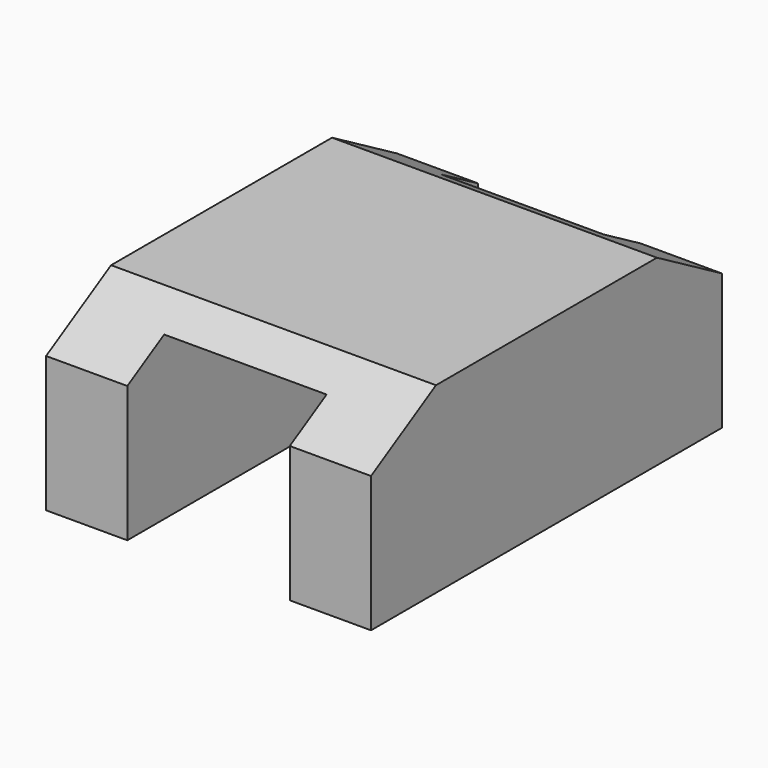
from build123d import *

# Parameters (mm, degrees)
F1_DEPTH    = 68.58
F2_T1_DEPTH = 116.511978168


# Not quite as in the source:
# - a fillet or chamfer that OpenCascade refuses, or shapes differently, is made with other operations: its cross-section is extruded or revolved along the edge and cut away or added


with BuildPart() as f1:
    # F0 (on Front) → F1 (new body)
    with BuildSketch(Plane.XZ):
        Polygon((-12.7, 0), (0, 0), (0, 28.575), (-50.8, 28.575), (-50.8, 0), (-38.1, 0), (-38.1, 25.4), (-12.7, 25.4), align=None)
    extrude(amount=F1_DEPTH)

    # F2: chamfer of 12.7 x 7.3323484187 on 2 edges, made by hand

    # F2_s2 → F2_t1 (cut)
    with BuildSketch(Plane.YZ.offset(-83.655989084)):
        Polygon((-12.7, 28.575), (0, 21.2426515813), (0, 28.575), align=None)
        Polygon((-55.88, 28.575), (-68.58, 21.2426515813), (-68.58, 28.575), align=None)
    extrude(amount=F2_T1_DEPTH, mode=Mode.SUBTRACT)


solid = f1.part
